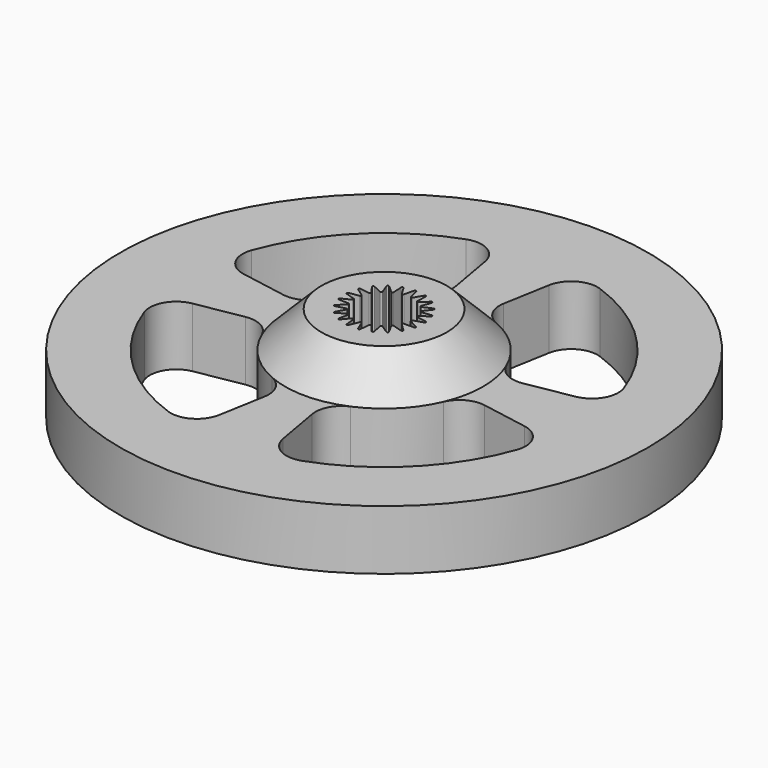
from build123d import *

# Parameters (mm, degrees)
F0_R     = 4.5
F1_DEPTH = 5
F2_R     = 20
F2_R_2   = 0.9
F3_DEPTH = 2.26
F4_R     = 3
F5_DEPTH = 1.7
F8_DEPTH = 1


# Not quite as in the source:
# - a fillet or chamfer that OpenCascade refuses, or shapes differently, is made with other operations: its cross-section is extruded or revolved along the edge and cut away or added


with BuildPart() as f1:
    # F0 (on Top) → F1 (new body)
    with BuildSketch(Plane.XY):
        Circle(F0_R)
        with BuildLine():
            ThreePointArc((-0.4050154324, 2.1915548193), (-0.3246414037, 2.1538549816), (-0.2589503899, 2.2135705822))
            Line((-0.2589503899, 2.2135705822), (-0.0776143951, 2.9393908656))
            ThreePointArc((-0.0776143951, 2.9393908656), (0, 3), (0.0776143951, 2.9393908656))
            Line((0.0776143951, 2.9393908656), (0.2589503899, 2.2135705822))
            ThreePointArc((0.2589503899, 2.2135705822), (0.3246414037, 2.1538549816), (0.4050154324, 2.1915548193))
            Line((0.4050154324, 2.1915548193), (0.7922344619, 2.8316792213))
            ThreePointArc((0.7922344619, 2.8316792213), (0.8842655232, 2.8667184174), (0.9405668726, 2.7859247321))
            Line((0.9405668726, 2.7859247321), (0.8999073336, 2.0389008847))
            ThreePointArc((0.8999073336, 2.0389008847), (0.9450783978, 1.9624755145), (1.0329938561, 1.9748097933))
            Line((1.0329938561, 1.9748097933), (1.5916898104, 2.4723604516))
            ThreePointArc((1.5916898104, 2.4723604516), (1.6899601742, 2.4787163229), (1.7199458558, 2.3849169604))
            Line((1.7199458558, 2.3849169604), (1.4609035616, 1.683065896))
            ThreePointArc((1.4609035616, 1.683065896), (1.4815410288, 1.5967214857), (1.5691862425, 1.5825942509))
            Line((1.5691862425, 1.5825942509), (2.2497165341, 1.893361606))
            ThreePointArc((2.2497165341, 1.893361606), (2.3454944474, 1.8704694056), (2.3465001018, 1.7719988508))
            Line((2.3465001018, 1.7719988508), (1.8920920971, 1.1776831165))
            ThreePointArc((1.8920920971, 1.1776831165), (1.8863622378, 1.0890917458), (1.965949545, 1.0497582641))
            Line((1.965949545, 1.0497582641), (2.7078460711, 1.1461292728))
            ThreePointArc((2.7078460711, 1.1461292728), (2.7926212459, 1.0960230731), (2.7645575164, 1.0016308669))
            Line((2.7645575164, 1.0016308669), (2.1551599464, 0.5676580238))
            ThreePointArc((2.1551599464, 0.5676580238), (2.1235718838, 0.4846914249), (2.188029603, 0.4236466488))
            Line((2.188029603, 0.4236466488), (2.9253716015, 0.297058324))
            ThreePointArc((2.9253716015, 0.297058324), (2.9916113915, 0.2241902808), (2.9369718636, 0.1422635849))
            Line((2.9369718636, 0.1422635849), (2.2267323767, -0.0928059753))
            ThreePointArc((2.2267323767, -0.0928059753), (2.1720928488, -0.1627758562), (2.2156936287, -0.2401078303))
            Line((2.2156936287, -0.2401078303), (2.8829650274, -0.5784075605))
            ThreePointArc((2.8829650274, -0.5784075605), (2.9247837365, -0.6675628019), (2.848423372, -0.7297444409))
            Line((2.848423372, -0.7297444409), (2.1004498635, -0.7450237563))
            ThreePointArc((2.1004498635, -0.7450237563), (2.027613832, -0.7957797881), (2.0464835522, -0.8825276751))
            Line((2.0464835522, -0.8825276751), (2.5843943588, -1.4024793949))
            ThreePointArc((2.5843943588, -1.4024793949), (2.5980762114, -1.5), (2.5067799637, -1.5369114707))
            Line((2.5067799637, -1.5369114707), (1.7875331623, -1.331042907))
            ThreePointArc((1.7875331623, -1.331042907), (1.7029724283, -1.3580751936), (1.6954344311, -1.446531063))
            Line((1.6954344311, -1.446531063), (2.0561889101, -2.1019347804))
            ThreePointArc((2.0561889101, -2.1019347804), (2.0405182133, -2.1991556155), (1.9423981548, -2.2075171717))
            Line((1.9423981548, -2.2075171717), (1.3157862951, -1.7987930543))
            ThreePointArc((1.3157862951, -1.7987930543), (1.2270144509, -1.7996996583), (1.1937385206, -1.882003818))
            Line((1.1937385206, -1.882003818), (1.3452820532, -2.6146240365))
            ThreePointArc((1.3452820532, -2.6146240365), (1.3016512174, -2.7029066037), (1.2054257458, -2.6819752845))
            Line((1.2054257458, -2.6819752845), (0.7271260414, -2.1067125448))
            ThreePointArc((0.7271260414, -2.1067125448), (0.642030855, -2.0814129106), (0.5859737039, -2.1502522747))
            Line((0.5859737039, -2.1502522747), (0.5148409823, -2.8949924729))
            ThreePointArc((0.5148409823, -2.8949924729), (0.4471267985, -2.9664924787), (0.3613459693, -2.9181281235))
            Line((0.3613459693, -2.9181281235), (0.0738574479, -2.2274413806))
            ThreePointArc((0.0738574479, -2.2274413806), (0, -2.1781834916), (-0.0738574479, -2.2274413806))
            Line((-0.0738574479, -2.2274413806), (-0.3613459693, -2.9181281235))
            ThreePointArc((-0.3613459693, -2.9181281235), (-0.4471267985, -2.9664924787), (-0.5148409823, -2.8949924729))
            Line((-0.5148409823, -2.8949924729), (-0.5859737039, -2.1502522747))
            ThreePointArc((-0.5859737039, -2.1502522747), (-0.642030855, -2.0814129106), (-0.7271260414, -2.1067125448))
            Line((-0.7271260414, -2.1067125448), (-1.2054257458, -2.6819752845))
            ThreePointArc((-1.2054257458, -2.6819752845), (-1.3016512174, -2.7029066037), (-1.3452820532, -2.6146240365))
            Line((-1.3452820532, -2.6146240365), (-1.1937385206, -1.882003818))
            ThreePointArc((-1.1937385206, -1.882003818), (-1.2270144509, -1.7996996583), (-1.3157862951, -1.7987930543))
            Line((-1.3157862951, -1.7987930543), (-1.9423981548, -2.2075171717))
            ThreePointArc((-1.9423981548, -2.2075171717), (-2.0405182133, -2.1991556155), (-2.0561889101, -2.1019347804))
            Line((-2.0561889101, -2.1019347804), (-1.6954344311, -1.446531063))
            ThreePointArc((-1.6954344311, -1.446531063), (-1.7029724283, -1.3580751936), (-1.7875331623, -1.331042907))
            Line((-1.7875331623, -1.331042907), (-2.5067799637, -1.5369114707))
            ThreePointArc((-2.5067799637, -1.5369114707), (-2.5980762114, -1.5), (-2.5843943588, -1.4024793949))
            Line((-2.5843943588, -1.4024793949), (-2.0464835522, -0.8825276751))
            ThreePointArc((-2.0464835522, -0.8825276751), (-2.027613832, -0.7957797881), (-2.1004498635, -0.7450237563))
            Line((-2.1004498635, -0.7450237563), (-2.848423372, -0.7297444409))
            ThreePointArc((-2.848423372, -0.7297444409), (-2.9247837365, -0.6675628019), (-2.8829650274, -0.5784075605))
            Line((-2.8829650274, -0.5784075605), (-2.2156936287, -0.2401078303))
            ThreePointArc((-2.2156936287, -0.2401078303), (-2.1720928488, -0.1627758562), (-2.2267323767, -0.0928059753))
            Line((-2.2267323767, -0.0928059753), (-2.9369718636, 0.1422635849))
            ThreePointArc((-2.9369718636, 0.1422635849), (-2.9916113915, 0.2241902808), (-2.9253716015, 0.297058324))
            Line((-2.9253716015, 0.297058324), (-2.188029603, 0.4236466488))
            ThreePointArc((-2.188029603, 0.4236466488), (-2.1235718838, 0.4846914249), (-2.1551599464, 0.5676580238))
            Line((-2.1551599464, 0.5676580238), (-2.7645575164, 1.0016308669))
            ThreePointArc((-2.7645575164, 1.0016308669), (-2.7926212459, 1.0960230731), (-2.7078460711, 1.1461292728))
            Line((-2.7078460711, 1.1461292728), (-1.965949545, 1.0497582641))
            ThreePointArc((-1.965949545, 1.0497582641), (-1.8863622378, 1.0890917458), (-1.8920920971, 1.1776831165))
            Line((-1.8920920971, 1.1776831165), (-2.3465001018, 1.7719988508))
            ThreePointArc((-2.3465001018, 1.7719988508), (-2.3454944474, 1.8704694056), (-2.2497165341, 1.893361606))
            Line((-2.2497165341, 1.893361606), (-1.5691862425, 1.5825942509))
            ThreePointArc((-1.5691862425, 1.5825942509), (-1.4815410288, 1.5967214857), (-1.4609035616, 1.683065896))
            Line((-1.4609035616, 1.683065896), (-1.7199458558, 2.3849169604))
            ThreePointArc((-1.7199458558, 2.3849169604), (-1.6899601742, 2.4787163229), (-1.5916898104, 2.4723604516))
            Line((-1.5916898104, 2.4723604516), (-1.0329938561, 1.9748097933))
            ThreePointArc((-1.0329938561, 1.9748097933), (-0.9450783978, 1.9624755145), (-0.8999073336, 2.0389008847))
            Line((-0.8999073336, 2.0389008847), (-0.9405668726, 2.7859247321))
            ThreePointArc((-0.9405668726, 2.7859247321), (-0.8842655232, 2.8667184174), (-0.7922344619, 2.8316792213))
            Line((-0.7922344619, 2.8316792213), (-0.4050154324, 2.1915548193))
        make_face(mode=Mode.SUBTRACT)
    extrude(amount=F1_DEPTH)

    # F2 (on Top) → F3 (join, symmetric)
    with BuildSketch(Plane.XY):
        Circle(F2_R)
        with BuildLine():
            ThreePointArc((-2.4229387374, -12.5827149104), (-3.3887522104, -13.9652686869), (-5.0683318193, -14.1177906405))
            ThreePointArc((-5.0683318193, -14.1177906405), (-10.6066017178, -10.6066017178), (-14.1177906405, -5.0683318193))
            ThreePointArc((-14.1177906405, -5.0683318193), (-13.9652686869, -3.3887522104), (-12.5827149104, -2.4229387374))
            Line((-12.5827149104, -2.4229387374), (-9.0661456358, -1.8028726948))
            ThreePointArc((-9.0661456358, -1.8028726948), (-7.7706307754, -2.0115561559), (-6.8833020635, -2.9782801585))
            ThreePointArc((-6.8833020635, -2.9782801585), (-5.3033008589, -5.3033008589), (-2.9782801585, -6.8833020635))
            ThreePointArc((-2.9782801585, -6.8833020635), (-2.0115561559, -7.7706307754), (-1.8028726948, -9.0661456358))
            Line((-1.8028726948, -9.0661456358), (-2.4229387374, -12.5827149104))
        make_face(mode=Mode.SUBTRACT)
        with BuildLine():
            Line((2.4229387374, -12.5827149104), (1.8028726948, -9.0661456358))
            ThreePointArc((1.8028726948, -9.0661456358), (2.0115561559, -7.7706307754), (2.9782801585, -6.8833020635))
            ThreePointArc((2.9782801585, -6.8833020635), (5.3033008589, -5.3033008589), (6.8833020635, -2.9782801585))
            ThreePointArc((6.8833020635, -2.9782801585), (7.7706307754, -2.0115561559), (9.0661456358, -1.8028726948))
            Line((9.0661456358, -1.8028726948), (12.5827149104, -2.4229387374))
            ThreePointArc((12.5827149104, -2.4229387374), (13.9652686869, -3.3887522104), (14.1177906405, -5.0683318193))
            ThreePointArc((14.1177906405, -5.0683318193), (10.6066017178, -10.6066017178), (5.0683318193, -14.1177906405))
            ThreePointArc((5.0683318193, -14.1177906405), (3.3887522104, -13.9652686869), (2.4229387374, -12.5827149104))
        make_face(mode=Mode.SUBTRACT)
        with BuildLine():
            ThreePointArc((-2.9782801585, 6.8833020635), (-5.3033008589, 5.3033008589), (-6.8833020635, 2.9782801585))
            ThreePointArc((-6.8833020635, 2.9782801585), (-7.7706307754, 2.0115561559), (-9.0661456358, 1.8028726948))
            Line((-9.0661456358, 1.8028726948), (-12.5827149104, 2.4229387374))
            ThreePointArc((-12.5827149104, 2.4229387374), (-13.9652686869, 3.3887522104), (-14.1177906405, 5.0683318193))
            ThreePointArc((-14.1177906405, 5.0683318193), (-10.6066017178, 10.6066017178), (-5.0683318193, 14.1177906405))
            ThreePointArc((-5.0683318193, 14.1177906405), (-3.3887522104, 13.9652686869), (-2.4229387374, 12.5827149104))
            Line((-2.4229387374, 12.5827149104), (-1.8028726948, 9.0661456358))
            ThreePointArc((-1.8028726948, 9.0661456358), (-2.0115561559, 7.7706307754), (-2.9782801585, 6.8833020635))
        make_face(mode=Mode.SUBTRACT)
        Circle(F2_R_2, mode=Mode.SUBTRACT)
        with BuildLine():
            ThreePointArc((9.0661456358, 1.8028726948), (7.7706307754, 2.0115561559), (6.8833020635, 2.9782801585))
            ThreePointArc((6.8833020635, 2.9782801585), (5.3033008589, 5.3033008589), (2.9782801585, 6.8833020635))
            ThreePointArc((2.9782801585, 6.8833020635), (2.0115561559, 7.7706307754), (1.8028726948, 9.0661456358))
            Line((1.8028726948, 9.0661456358), (2.4229387374, 12.5827149104))
            ThreePointArc((2.4229387374, 12.5827149104), (3.3887522104, 13.9652686869), (5.0683318193, 14.1177906405))
            ThreePointArc((5.0683318193, 14.1177906405), (10.6066017178, 10.6066017178), (14.1177906405, 5.0683318193))
            ThreePointArc((14.1177906405, 5.0683318193), (13.9652686869, 3.3887522104), (12.5827149104, 2.4229387374))
            Line((12.5827149104, 2.4229387374), (9.0661456358, 1.8028726948))
        make_face(mode=Mode.SUBTRACT)
    extrude(amount=F3_DEPTH, both=True)

    # F4 (on face) → F5 (cut)
    with BuildSketch(Plane(origin=(0, 0, -2.26), x_dir=(1, 0, 0), z_dir=(0, 0, -1))):
        Circle(F4_R)
    extrude(amount=-F5_DEPTH, mode=Mode.SUBTRACT)

    # F7: chamfer of 3 on 1 edges, made by hand


with BuildPart() as f7_tool2:
    # F7_s3 → F7_t4 (revolve)
    with BuildSketch(Plane.XZ):
        Polygon((4.5, 5.26), (7.5, 2.26), (4.5, 2.26), align=None)
    revolve(axis=Axis((0, 0, 2.26), (0, 0, -1)))

    split(bisect_by=Plane.XY.offset(5), keep=Keep.BOTTOM)


with BuildPart() as f1_1:
    add(f1.part)

    # F7_t1: union F7_tool2
    add(f7_tool2.part)

    # F8 (cut): a face of the model
    f8_faces = [f1_1.faces().sort_by_distance(p)[0] for p in [
        (-1.9445548766, 1.6611069614, 2.26),
    ]]
    extrude(f8_faces, amount=-F8_DEPTH, mode=Mode.SUBTRACT)


solid = f1_1.part
